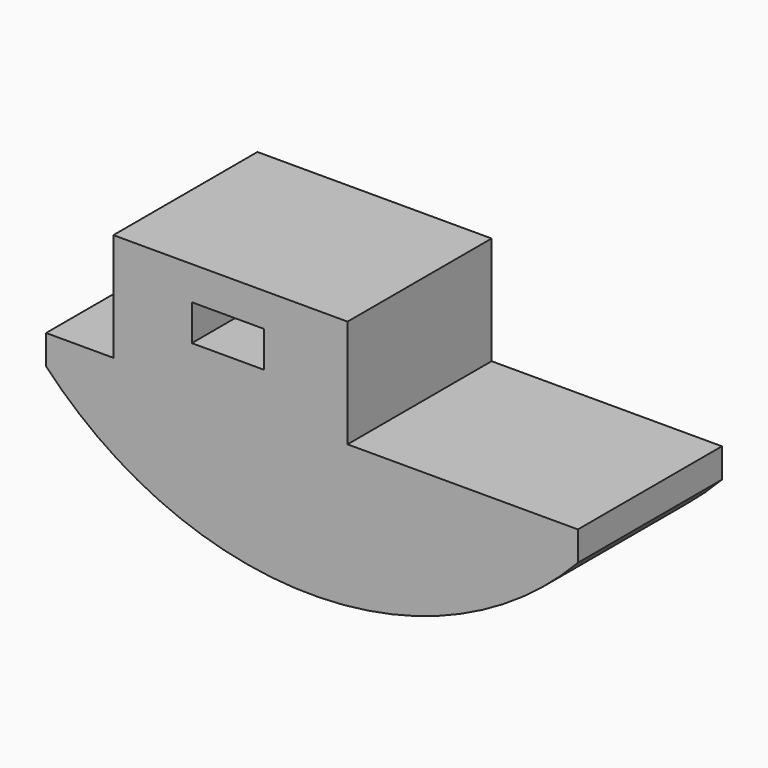
from build123d import *

# Parameters (mm, degrees)
F1_DEPTH = 127
F0_W     = 50.8
F0_H     = 25.4
F2_START = 36.322
F0_W_2   = 37.3759667383
F0_H_2   = 15.9422476888
F2_DEPTH = 24.638


# Not quite as in the source:
# - a feature names something its author has since deleted; it is built from what else it names


with BuildPart() as f1:
    # F0 (on Front) → F1 (new body)
    with BuildSketch(Plane.XZ):
        Polygon((-307.3281569301, -41.3140561762), (-306.4012624873, -41.288353515), (-306.7446031917, -40.692556251), align=None)
    extrude(amount=F1_DEPTH)


with BuildPart() as f1b:
    # F0 (on Front) → F1, piece 2 (new body)
    with BuildSketch(Plane.XZ):
        with BuildLine():
            Line((-21.9041593159, -73.2302481236), (-146.6470350679, -73.2302481236))
            ThreePointArc((-146.6470350679, -73.2302481236), (-84.2755971919, -80.8868076681), (-21.9041593159, -73.2302481236))
        make_face()
        Polygon((-224.3537551874, 96.9131923319), (-224.3537551874, 20.7131923319), (-197.7432811606, 20.7131923319), (-83.9606040237, 20.7131923319), (-59.1853400261, 20.7131923319), (-59.1853400261, 96.9131923319), (-160.1215863499, 96.9131923319), (-161.9567914552, 96.9131923319), align=None)
        with Locations((-143.6194745734, 60.5380154436)):
            Rectangle(F0_W, F0_H, mode=Mode.SUBTRACT)
        with BuildLine():
            Line((-224.3537551874, 20.7131923319), (-271.8233303091, 20.7131923319))
            Line((-271.8233303091, 20.7131923319), (-271.8233303091, 0))
            ThreePointArc((-271.8233303091, 0), (-214.4891345739, -45.5959789578), (-146.6470350679, -73.2302481236))
            Line((-146.6470350679, -73.2302481236), (-21.9041593159, -73.2302481236))
            ThreePointArc((-21.9041593159, -73.2302481236), (45.9379401902, -45.5959789578), (103.2721359253, 0))
            Line((103.2721359253, 0), (103.2721359253, 20.7131923319))
            Line((103.2721359253, 20.7131923319), (-59.1853400261, 20.7131923319))
            Line((-59.1853400261, 20.7131923319), (-83.9606040237, 20.7131923319))
            Line((-83.9606040237, 20.7131923319), (-197.7432811606, 20.7131923319))
            Line((-197.7432811606, 20.7131923319), (-224.3537551874, 20.7131923319))
        make_face()
    extrude(amount=F1_DEPTH)


with BuildPart() as f2:
    # F0 (on Front) → F2 (new body)
    with BuildSketch(Plane.XZ.offset(F2_START)):
        with Locations((-253.13534694, -42.8495634074)):
            Rectangle(F0_W_2, F0_H_2)
        Polygon((-271.8233303091, -50.8206872518), (-271.8233303091, -34.8784395629), (-284.9155039664, -34.8784395629), (-284.9155039664, -40.692556251), (-284.9155039664, -50.8206872518), align=None)
    extrude(amount=F2_DEPTH)


solid = Compound([f1b.part, f2.part])
